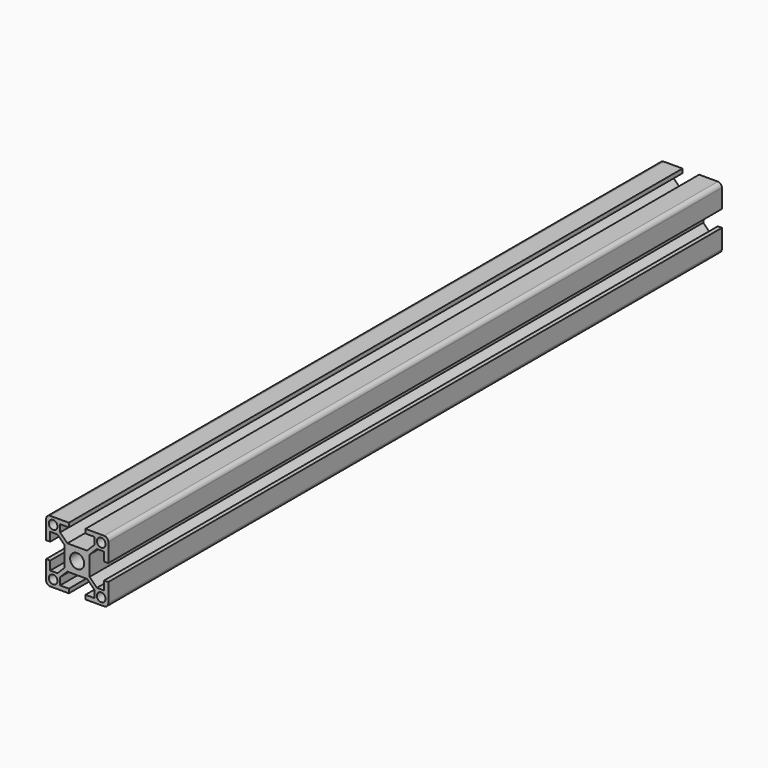
from build123d import *

# Parameters (mm, degrees)
F1_DEPTH = 370
F2_DEPTH = 400
F3_W     = 18.6485039899
F3_H     = 8
F3_W_2   = 19.9612321942
F3_R     = 3.4
F3_R_2   = 2.1
F4_DEPTH = 370
F5_R     = 2


# Not quite as in the source:
# - a pattern or mirror of a feature is missing from the dataset's text; its kind, count and spacing are read off the source's solid


with BuildPart() as f1:
    # F0 (on Front) → F1 (new body)
    with BuildSketch(Plane.XZ):
        Polygon((15, -15), (15, 15), (4, 15), (4, 13), (8.25, 13), (8.25, 9.5), (4.75, 6), (-4.75, 6), (-8.25, 9.5), (-8.25, 13), (-4, 13), (-4, 15), (-15, 15), (-15, -15), align=None)
        Polygon((4, 13), (4, 15), (-4, 15), (-4, 13), (-8.25, 13), (-8.25, 9.5), (-4.75, 6), (4.75, 6), (8.25, 9.5), (8.25, 13), align=None)
    extrude(amount=F1_DEPTH)

    # F0 (on Front) → F2 (cut)
    with BuildSketch(Plane.XZ):
        Polygon((4, 13), (4, 15), (-4, 15), (-4, 13), (-8.25, 13), (-8.25, 9.5), (-4.75, 6), (4.75, 6), (8.25, 9.5), (8.25, 13), align=None)
    f2 = extrude(amount=F2_DEPTH, mode=Mode.SUBTRACT)

    # F2_copies: F2 across plane
    add(f2.mirror(Plane(origin=(0, 0, 0), x_dir=(-1, 0, 0), z_dir=(0, 0, -1))), mode=Mode.SUBTRACT)

    # F3 (on face) → F4 (cut)
    with BuildSketch(Plane(origin=(0, 0, 0), x_dir=(-1, 0, 0), z_dir=(0, 1, 0))):
        Polygon((-6, 4.75), (-9.5, 8.25), (-13, 8.25), (-13, 4), (-13, -4), (-13, -8.25), (-9.5, -8.25), (-6, -4.75), align=None)
        with Locations((-22.3242519949, 0)):
            Rectangle(F3_W, F3_H)
        Polygon((13, 8.25), (9.5, 8.25), (6, 4.75), (6, -4.75), (9.5, -8.25), (13, -8.25), (13, -4), (13, 4), align=None)
        with Locations((22.9806160971, 0)):
            Rectangle(F3_W_2, F3_H)
        Circle(F3_R)
        with Locations((-11.6, 11.6)):
            Circle(F3_R_2)
        with Locations((-11.6, -11.6)):
            Circle(F3_R_2)
        with Locations((11.6, -11.6)):
            Circle(F3_R_2)
        with Locations((11.6, 11.6)):
            Circle(F3_R_2)
    extrude(amount=-F4_DEPTH, mode=Mode.SUBTRACT)

    # F5
    f5_edges = [f1.edges().sort_by_distance(p)[0] for p in [
        (-15, -185, 15),
        (-15, -185, -15),
        (15, -185, -15),
        (15, -185, 15),
    ]]
    fillet(f5_edges, radius=F5_R)


solid = f1.part
